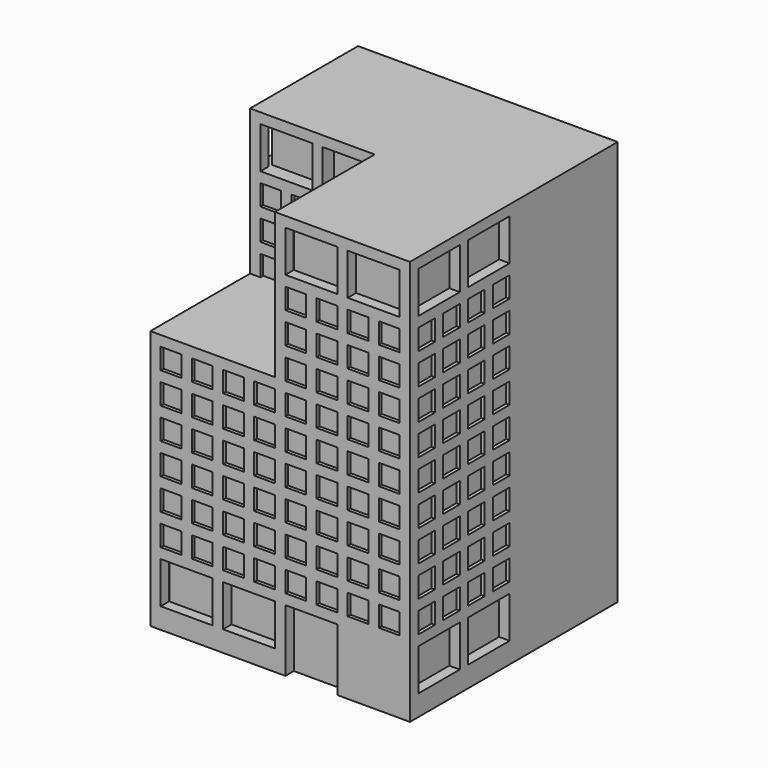
from build123d import *

# Parameters (mm, degrees)
F1_DEPTH     = 469.9
F2_W         = 225.552
F2_H         = 244.348
F3_DEPTH     = 281.94
F4_W         = 93.98
F4_H         = 75.184
F5_DEPTH     = 19.05
F4_W_2       = 37.592
F4_H_2       = 37.592
F6_DEPTH     = 6.35
F7_W         = 93.98
F7_H         = 75.184
F8_DEPTH     = 19.05
F7_W_2       = 187.96
F7_H_2       = 244.348
F7_W_3       = 37.592
F7_H_3       = 37.592
F9_DEPTH     = 6.35
F10_W        = 93.98
F10_H        = 75.184
F11_DEPTH    = 19.05
F10_W_2      = 37.592
F10_H_2      = 37.592
F12_DEPTH    = 6.35
F13_W        = 93.98
F13_H        = 75.184
F14_DEPTH    = 19.05
F13_W_2      = 37.592
F13_H_2      = 37.592
F13_W_3      = 187.96
F13_H_3      = 244.348
F15_DEPTH    = 6.35
F16_W        = 93.98
F16_H        = 75.184
F17_DEPTH    = 19.05
F16_W_2      = 37.592
F16_H_2      = 37.592
F18_DEPTH    = 6.35
F19_W        = 93.98
F19_H        = 75.184
F20_DEPTH    = 19.05
F21_DEPTH    = 224.028
F22_DEPTH    = 223.52
F19_W_2      = 37.592
F19_H_2      = 37.592
F20_FACE_W   = 93.726
F20_FACE_H   = 75.184
F20_FACE_W_2 = 93.98
F23_DEPTH    = 6.35
F24_DEPTH    = 18.796
F25_DEPTH    = 18.796


with BuildPart() as f1:
    # F0 (on Front) → F1 (new body)
    with BuildSketch(Plane.XZ):
        Polygon((109.2016026378, 21.9071136281), (109.2016026378, -466.788886372), (579.1016026378, -466.788886372), (579.1016026378, 303.847113628), (334.7536026378, 303.847113628), (334.7536026378, 21.9071136281), align=None)
    extrude(amount=F1_DEPTH)

    # F2 (on face) → F3 (join)
    with BuildSketch(Plane.XY.offset(21.907113628)):
        with Locations((221.9776026378, -122.174)):
            Rectangle(F2_W, F2_H)
    extrude(amount=F3_DEPTH)

    # F4 (on face) → F5 (cut)
    with BuildSketch(Plane.XZ.offset(469.9)):
        with Locations((400.5396026378, 228.663113628)):
            Rectangle(F4_W, F4_H)
        with Locations((513.3156026378, 228.663113628)):
            Rectangle(F4_W, F4_H)
        Polygon((447.5296026378, -335.216886372), (353.5496026378, -335.216886372), (353.5496026378, -410.400886372), (353.5496026378, -466.788886372), (447.5296026378, -466.788886372), (447.5296026378, -410.400886372), align=None)
        with Locations((287.7636026378, -372.808886372)):
            Rectangle(F4_W, F4_H)
        with Locations((174.9876026378, -372.808886372)):
            Rectangle(F4_W, F4_H)
    extrude(amount=-F5_DEPTH, mode=Mode.SUBTRACT)

    # F4 (on face) → F6 (cut)
    with BuildSketch(Plane.XZ.offset(469.9)):
        with Locations((174.9876026378, -372.808886372)):
            Rectangle(F4_W, F4_H)
        with Locations((287.7636026378, -372.808886372)):
            Rectangle(F4_W, F4_H)
        with Locations((541.5096026378, -297.624886372)):
            Rectangle(F4_W_2, F4_H_2)
        with Locations((541.5096026378, -241.236886372)):
            Rectangle(F4_W_2, F4_H_2)
        with Locations((541.5096026378, -184.848886372)):
            Rectangle(F4_W_2, F4_H_2)
        with Locations((541.5096026378, -128.460886372)):
            Rectangle(F4_W_2, F4_H_2)
        with Locations((541.5096026378, -72.072886372)):
            Rectangle(F4_W_2, F4_H_2)
        with Locations((541.5096026378, -15.684886372)):
            Rectangle(F4_W_2, F4_H_2)
        with Locations((485.1216026378, -297.624886372)):
            Rectangle(F4_W_2, F4_H_2)
        with Locations((485.1216026378, -241.236886372)):
            Rectangle(F4_W_2, F4_H_2)
        with Locations((485.1216026378, -184.848886372)):
            Rectangle(F4_W_2, F4_H_2)
        with Locations((485.1216026378, -128.460886372)):
            Rectangle(F4_W_2, F4_H_2)
        with Locations((485.1216026378, -72.072886372)):
            Rectangle(F4_W_2, F4_H_2)
        with Locations((485.1216026378, -15.684886372)):
            Rectangle(F4_W_2, F4_H_2)
        with Locations((428.7336026378, -297.624886372)):
            Rectangle(F4_W_2, F4_H_2)
        with Locations((428.7336026378, -241.236886372)):
            Rectangle(F4_W_2, F4_H_2)
        with Locations((428.7336026378, -184.848886372)):
            Rectangle(F4_W_2, F4_H_2)
        with Locations((428.7336026378, -128.460886372)):
            Rectangle(F4_W_2, F4_H_2)
        with Locations((428.7336026378, -72.072886372)):
            Rectangle(F4_W_2, F4_H_2)
        with Locations((428.7336026378, -15.684886372)):
            Rectangle(F4_W_2, F4_H_2)
        with Locations((372.3456026378, -297.624886372)):
            Rectangle(F4_W_2, F4_H_2)
        with Locations((372.3456026378, -241.236886372)):
            Rectangle(F4_W_2, F4_H_2)
        with Locations((372.3456026378, -184.848886372)):
            Rectangle(F4_W_2, F4_H_2)
        with Locations((372.3456026378, -128.460886372)):
            Rectangle(F4_W_2, F4_H_2)
        with Locations((372.3456026378, -72.072886372)):
            Rectangle(F4_W_2, F4_H_2)
        with Locations((372.3456026378, -15.684886372)):
            Rectangle(F4_W_2, F4_H_2)
        with Locations((315.9576026378, -297.624886372)):
            Rectangle(F4_W_2, F4_H_2)
        with Locations((315.9576026378, -241.236886372)):
            Rectangle(F4_W_2, F4_H_2)
        with Locations((315.9576026378, -184.848886372)):
            Rectangle(F4_W_2, F4_H_2)
        with Locations((315.9576026378, -128.460886372)):
            Rectangle(F4_W_2, F4_H_2)
        with Locations((315.9576026378, -72.072886372)):
            Rectangle(F4_W_2, F4_H_2)
        with Locations((315.9576026378, -15.684886372)):
            Rectangle(F4_W_2, F4_H_2)
        with Locations((259.5696026378, -297.624886372)):
            Rectangle(F4_W_2, F4_H_2)
        with Locations((259.5696026378, -241.236886372)):
            Rectangle(F4_W_2, F4_H_2)
        with Locations((259.5696026378, -184.848886372)):
            Rectangle(F4_W_2, F4_H_2)
        with Locations((259.5696026378, -128.460886372)):
            Rectangle(F4_W_2, F4_H_2)
        with Locations((259.5696026378, -72.072886372)):
            Rectangle(F4_W_2, F4_H_2)
        with Locations((259.5696026378, -15.684886372)):
            Rectangle(F4_W_2, F4_H_2)
        with Locations((203.1816026378, -297.624886372)):
            Rectangle(F4_W_2, F4_H_2)
        with Locations((203.1816026378, -241.236886372)):
            Rectangle(F4_W_2, F4_H_2)
        with Locations((203.1816026378, -184.848886372)):
            Rectangle(F4_W_2, F4_H_2)
        with Locations((203.1816026378, -128.460886372)):
            Rectangle(F4_W_2, F4_H_2)
        with Locations((203.1816026378, -72.072886372)):
            Rectangle(F4_W_2, F4_H_2)
        with Locations((203.1816026378, -15.684886372)):
            Rectangle(F4_W_2, F4_H_2)
        with Locations((146.7936026378, -297.624886372)):
            Rectangle(F4_W_2, F4_H_2)
        with Locations((146.7936026378, -241.236886372)):
            Rectangle(F4_W_2, F4_H_2)
        with Locations((146.7936026378, -184.848886372)):
            Rectangle(F4_W_2, F4_H_2)
        with Locations((146.7936026378, -128.460886372)):
            Rectangle(F4_W_2, F4_H_2)
        with Locations((146.7936026378, -72.072886372)):
            Rectangle(F4_W_2, F4_H_2)
        with Locations((146.7936026378, -15.684886372)):
            Rectangle(F4_W_2, F4_H_2)
        with Locations((513.3156026378, 228.663113628)):
            Rectangle(F4_W, F4_H)
        with Locations((400.5396026378, 228.663113628)):
            Rectangle(F4_W, F4_H)
        with Locations((541.5096026378, 40.703113628)):
            Rectangle(F4_W_2, F4_H_2)
        with Locations((541.5096026378, 97.091113628)):
            Rectangle(F4_W_2, F4_H_2)
        with Locations((541.5096026378, 153.479113628)):
            Rectangle(F4_W_2, F4_H_2)
        with Locations((485.1216026378, 40.703113628)):
            Rectangle(F4_W_2, F4_H_2)
        with Locations((485.1216026378, 97.091113628)):
            Rectangle(F4_W_2, F4_H_2)
        with Locations((485.1216026378, 153.479113628)):
            Rectangle(F4_W_2, F4_H_2)
        with Locations((428.7336026378, 40.703113628)):
            Rectangle(F4_W_2, F4_H_2)
        with Locations((428.7336026378, 97.091113628)):
            Rectangle(F4_W_2, F4_H_2)
        with Locations((428.7336026378, 153.479113628)):
            Rectangle(F4_W_2, F4_H_2)
        with Locations((372.3456026378, 40.703113628)):
            Rectangle(F4_W_2, F4_H_2)
        with Locations((372.3456026378, 97.091113628)):
            Rectangle(F4_W_2, F4_H_2)
        with Locations((372.3456026378, 153.479113628)):
            Rectangle(F4_W_2, F4_H_2)
    extrude(amount=-F6_DEPTH, mode=Mode.SUBTRACT)

    # F7 (on face) → F8 (cut)
    with BuildSketch(Plane(origin=(0, 0, 0), x_dir=(-1, 0, 0), z_dir=(0, 1, 0))):
        with Locations((-400.5396026378, 228.663113628)):
            Rectangle(F7_W, F7_H)
        with Locations((-287.7636026378, 228.663113628)):
            Rectangle(F7_W, F7_H)
        with Locations((-174.9876026378, 228.663113628)):
            Rectangle(F7_W, F7_H)
        with Locations((-400.5396026378, -372.8088863719)):
            Rectangle(F7_W, F7_H)
    extrude(amount=-F8_DEPTH, mode=Mode.SUBTRACT)

    # F7 (on face) → F9 (cut)
    with BuildSketch(Plane(origin=(0, 0, 0), x_dir=(-1, 0, 0), z_dir=(0, 1, 0))):
        with Locations((-240.7736026378, -344.614886372)):
            Rectangle(F7_W_2, F7_H_2)
        with Locations((-400.5396026378, -372.8088863719)):
            Rectangle(F7_W, F7_H)
        with Locations((-174.9876026378, 228.663113628)):
            Rectangle(F7_W, F7_H)
        with Locations((-287.7636026378, 228.663113628)):
            Rectangle(F7_W, F7_H)
        with Locations((-400.5396026378, 228.663113628)):
            Rectangle(F7_W, F7_H)
        with Locations((-146.7936026378, 153.479113628)):
            Rectangle(F7_W_3, F7_H_3)
        with Locations((-146.7936026378, 97.091113628)):
            Rectangle(F7_W_3, F7_H_3)
        with Locations((-146.7936026378, 40.703113628)):
            Rectangle(F7_W_3, F7_H_3)
        with Locations((-146.7936026378, -15.684886372)):
            Rectangle(F7_W_3, F7_H_3)
        with Locations((-146.7936026378, -72.072886372)):
            Rectangle(F7_W_3, F7_H_3)
        with Locations((-146.7936026378, -128.460886372)):
            Rectangle(F7_W_3, F7_H_3)
        with Locations((-146.7936026378, -184.848886372)):
            Rectangle(F7_W_3, F7_H_3)
        with Locations((-203.1816026378, 153.479113628)):
            Rectangle(F7_W_3, F7_H_3)
        with Locations((-203.1816026378, 97.091113628)):
            Rectangle(F7_W_3, F7_H_3)
        with Locations((-203.1816026378, 40.703113628)):
            Rectangle(F7_W_3, F7_H_3)
        with Locations((-203.1816026378, -15.684886372)):
            Rectangle(F7_W_3, F7_H_3)
        with Locations((-203.1816026378, -72.072886372)):
            Rectangle(F7_W_3, F7_H_3)
        with Locations((-203.1816026378, -128.460886372)):
            Rectangle(F7_W_3, F7_H_3)
        with Locations((-203.1816026378, -184.848886372)):
            Rectangle(F7_W_3, F7_H_3)
        with Locations((-259.5696026378, 153.479113628)):
            Rectangle(F7_W_3, F7_H_3)
        with Locations((-259.5696026378, 97.091113628)):
            Rectangle(F7_W_3, F7_H_3)
        with Locations((-259.5696026378, 40.703113628)):
            Rectangle(F7_W_3, F7_H_3)
        with Locations((-259.5696026378, -15.684886372)):
            Rectangle(F7_W_3, F7_H_3)
        with Locations((-259.5696026378, -72.072886372)):
            Rectangle(F7_W_3, F7_H_3)
        with Locations((-259.5696026378, -128.460886372)):
            Rectangle(F7_W_3, F7_H_3)
        with Locations((-259.5696026378, -184.848886372)):
            Rectangle(F7_W_3, F7_H_3)
        with Locations((-315.9576026378, 153.479113628)):
            Rectangle(F7_W_3, F7_H_3)
        with Locations((-315.9576026378, 97.091113628)):
            Rectangle(F7_W_3, F7_H_3)
        with Locations((-315.9576026378, 40.703113628)):
            Rectangle(F7_W_3, F7_H_3)
        with Locations((-315.9576026378, -15.684886372)):
            Rectangle(F7_W_3, F7_H_3)
        with Locations((-315.9576026378, -72.072886372)):
            Rectangle(F7_W_3, F7_H_3)
        with Locations((-315.9576026378, -128.460886372)):
            Rectangle(F7_W_3, F7_H_3)
        with Locations((-315.9576026378, -184.848886372)):
            Rectangle(F7_W_3, F7_H_3)
        with Locations((-372.3456026378, 153.479113628)):
            Rectangle(F7_W_3, F7_H_3)
        with Locations((-372.3456026378, 97.091113628)):
            Rectangle(F7_W_3, F7_H_3)
        with Locations((-372.3456026378, 40.703113628)):
            Rectangle(F7_W_3, F7_H_3)
        with Locations((-372.3456026378, -15.684886372)):
            Rectangle(F7_W_3, F7_H_3)
        with Locations((-372.3456026378, -72.072886372)):
            Rectangle(F7_W_3, F7_H_3)
        with Locations((-372.3456026378, -128.460886372)):
            Rectangle(F7_W_3, F7_H_3)
        with Locations((-372.3456026378, -184.848886372)):
            Rectangle(F7_W_3, F7_H_3)
        with Locations((-372.3456026378, -241.236886372)):
            Rectangle(F7_W_3, F7_H_3)
        with Locations((-372.3456026378, -297.624886372)):
            Rectangle(F7_W_3, F7_H_3)
        with Locations((-428.7336026378, 153.479113628)):
            Rectangle(F7_W_3, F7_H_3)
        with Locations((-428.7336026378, 97.091113628)):
            Rectangle(F7_W_3, F7_H_3)
        with Locations((-428.7336026378, 40.703113628)):
            Rectangle(F7_W_3, F7_H_3)
        with Locations((-428.7336026378, -15.684886372)):
            Rectangle(F7_W_3, F7_H_3)
        with Locations((-428.7336026378, -72.072886372)):
            Rectangle(F7_W_3, F7_H_3)
        with Locations((-428.7336026378, -128.460886372)):
            Rectangle(F7_W_3, F7_H_3)
        with Locations((-428.7336026378, -184.848886372)):
            Rectangle(F7_W_3, F7_H_3)
        with Locations((-428.7336026378, -241.236886372)):
            Rectangle(F7_W_3, F7_H_3)
        with Locations((-428.7336026378, -297.624886372)):
            Rectangle(F7_W_3, F7_H_3)
    extrude(amount=-F9_DEPTH, mode=Mode.SUBTRACT)

    # F10 (on face) → F11 (cut)
    with BuildSketch(Plane.YZ.offset(579.1016026378)):
        with Locations((-291.338, -372.808886372)):
            Rectangle(F10_W, F10_H)
        with Locations((-404.114, -372.808886372)):
            Rectangle(F10_W, F10_H)
        with Locations((-404.114, 228.663113628)):
            Rectangle(F10_W, F10_H)
        with Locations((-291.338, 228.663113628)):
            Rectangle(F10_W, F10_H)
    extrude(amount=-F11_DEPTH, mode=Mode.SUBTRACT)

    # F10 (on face) → F12 (cut)
    with BuildSketch(Plane.YZ.offset(579.1016026378)):
        with Locations((-432.308, -297.624886372)):
            Rectangle(F10_W_2, F10_H_2)
        with Locations((-432.308, -241.236886372)):
            Rectangle(F10_W_2, F10_H_2)
        with Locations((-432.308, -184.848886372)):
            Rectangle(F10_W_2, F10_H_2)
        with Locations((-432.308, -128.460886372)):
            Rectangle(F10_W_2, F10_H_2)
        with Locations((-432.308, -72.072886372)):
            Rectangle(F10_W_2, F10_H_2)
        with Locations((-432.308, -15.684886372)):
            Rectangle(F10_W_2, F10_H_2)
        with Locations((-432.308, 40.703113628)):
            Rectangle(F10_W_2, F10_H_2)
        with Locations((-432.308, 97.091113628)):
            Rectangle(F10_W_2, F10_H_2)
        with Locations((-432.308, 153.479113628)):
            Rectangle(F10_W_2, F10_H_2)
        with Locations((-375.92, -297.624886372)):
            Rectangle(F10_W_2, F10_H_2)
        with Locations((-375.92, -241.236886372)):
            Rectangle(F10_W_2, F10_H_2)
        with Locations((-375.92, -184.848886372)):
            Rectangle(F10_W_2, F10_H_2)
        with Locations((-375.92, -128.460886372)):
            Rectangle(F10_W_2, F10_H_2)
        with Locations((-375.92, -72.072886372)):
            Rectangle(F10_W_2, F10_H_2)
        with Locations((-375.92, -15.684886372)):
            Rectangle(F10_W_2, F10_H_2)
        with Locations((-375.92, 40.703113628)):
            Rectangle(F10_W_2, F10_H_2)
        with Locations((-375.92, 97.091113628)):
            Rectangle(F10_W_2, F10_H_2)
        with Locations((-375.92, 153.479113628)):
            Rectangle(F10_W_2, F10_H_2)
        with Locations((-319.532, -297.624886372)):
            Rectangle(F10_W_2, F10_H_2)
        with Locations((-319.532, -241.236886372)):
            Rectangle(F10_W_2, F10_H_2)
        with Locations((-319.532, -184.848886372)):
            Rectangle(F10_W_2, F10_H_2)
        with Locations((-319.532, -128.460886372)):
            Rectangle(F10_W_2, F10_H_2)
        with Locations((-319.532, -72.072886372)):
            Rectangle(F10_W_2, F10_H_2)
        with Locations((-319.532, -15.684886372)):
            Rectangle(F10_W_2, F10_H_2)
        with Locations((-319.532, 40.703113628)):
            Rectangle(F10_W_2, F10_H_2)
        with Locations((-319.532, 97.091113628)):
            Rectangle(F10_W_2, F10_H_2)
        with Locations((-319.532, 153.479113628)):
            Rectangle(F10_W_2, F10_H_2)
        with Locations((-263.144, -297.624886372)):
            Rectangle(F10_W_2, F10_H_2)
        with Locations((-263.144, -241.236886372)):
            Rectangle(F10_W_2, F10_H_2)
        with Locations((-263.144, -184.848886372)):
            Rectangle(F10_W_2, F10_H_2)
        with Locations((-263.144, -128.460886372)):
            Rectangle(F10_W_2, F10_H_2)
        with Locations((-263.144, -72.072886372)):
            Rectangle(F10_W_2, F10_H_2)
        with Locations((-263.144, -15.684886372)):
            Rectangle(F10_W_2, F10_H_2)
        with Locations((-263.144, 40.703113628)):
            Rectangle(F10_W_2, F10_H_2)
        with Locations((-263.144, 97.091113628)):
            Rectangle(F10_W_2, F10_H_2)
        with Locations((-263.144, 153.479113628)):
            Rectangle(F10_W_2, F10_H_2)
        with Locations((-291.338, 228.663113628)):
            Rectangle(F10_W, F10_H)
        with Locations((-404.114, 228.663113628)):
            Rectangle(F10_W, F10_H)
        with Locations((-404.114, -372.808886372)):
            Rectangle(F10_W, F10_H)
        with Locations((-291.338, -372.808886372)):
            Rectangle(F10_W, F10_H)
    extrude(amount=-F12_DEPTH, mode=Mode.SUBTRACT)

    # F13 (on face) → F14 (cut)
    with BuildSketch(Plane(origin=(109.2016026378, 0, 0), x_dir=(0, -1, 0), z_dir=(-1, 0, 0))):
        with Locations((65.786, 228.663113628)):
            Rectangle(F13_W, F13_H)
        with Locations((178.562, 228.663113628)):
            Rectangle(F13_W, F13_H)
        with Locations((291.338, -372.808886372)):
            Rectangle(F13_W, F13_H)
        with Locations((404.114, -372.808886372)):
            Rectangle(F13_W, F13_H)
    extrude(amount=-F14_DEPTH, mode=Mode.SUBTRACT)

    # F13 (on face) → F15 (cut)
    with BuildSketch(Plane(origin=(109.2016026378, 0, 0), x_dir=(0, -1, 0), z_dir=(-1, 0, 0))):
        with Locations((65.786, 228.663113628)):
            Rectangle(F13_W, F13_H)
        with Locations((178.562, 228.663113628)):
            Rectangle(F13_W, F13_H)
        with Locations((37.592, 153.479113628)):
            Rectangle(F13_W_2, F13_H_2)
        with Locations((37.592, 97.091113628)):
            Rectangle(F13_W_2, F13_H_2)
        with Locations((37.592, 40.703113628)):
            Rectangle(F13_W_2, F13_H_2)
        with Locations((37.592, -15.684886372)):
            Rectangle(F13_W_2, F13_H_2)
        with Locations((37.592, -72.072886372)):
            Rectangle(F13_W_2, F13_H_2)
        with Locations((37.592, -128.460886372)):
            Rectangle(F13_W_2, F13_H_2)
        with Locations((37.592, -184.848886372)):
            Rectangle(F13_W_2, F13_H_2)
        with Locations((93.98, 153.479113628)):
            Rectangle(F13_W_2, F13_H_2)
        with Locations((93.98, 97.091113628)):
            Rectangle(F13_W_2, F13_H_2)
        with Locations((93.98, 40.703113628)):
            Rectangle(F13_W_2, F13_H_2)
        with Locations((93.98, -15.684886372)):
            Rectangle(F13_W_2, F13_H_2)
        with Locations((93.98, -72.072886372)):
            Rectangle(F13_W_2, F13_H_2)
        with Locations((93.98, -128.460886372)):
            Rectangle(F13_W_2, F13_H_2)
        with Locations((93.98, -184.848886372)):
            Rectangle(F13_W_2, F13_H_2)
        with Locations((150.368, 153.479113628)):
            Rectangle(F13_W_2, F13_H_2)
        with Locations((150.368, 97.091113628)):
            Rectangle(F13_W_2, F13_H_2)
        with Locations((150.368, 40.703113628)):
            Rectangle(F13_W_2, F13_H_2)
        with Locations((150.368, -15.684886372)):
            Rectangle(F13_W_2, F13_H_2)
        with Locations((150.368, -72.072886372)):
            Rectangle(F13_W_2, F13_H_2)
        with Locations((150.368, -128.460886372)):
            Rectangle(F13_W_2, F13_H_2)
        with Locations((150.368, -184.848886372)):
            Rectangle(F13_W_2, F13_H_2)
        with Locations((206.756, 153.479113628)):
            Rectangle(F13_W_2, F13_H_2)
        with Locations((206.756, 97.091113628)):
            Rectangle(F13_W_2, F13_H_2)
        with Locations((206.756, 40.703113628)):
            Rectangle(F13_W_2, F13_H_2)
        with Locations((206.756, -15.684886372)):
            Rectangle(F13_W_2, F13_H_2)
        with Locations((206.756, -72.072886372)):
            Rectangle(F13_W_2, F13_H_2)
        with Locations((206.756, -128.460886372)):
            Rectangle(F13_W_2, F13_H_2)
        with Locations((206.756, -184.848886372)):
            Rectangle(F13_W_2, F13_H_2)
        with Locations((263.144, -15.684886372)):
            Rectangle(F13_W_2, F13_H_2)
        with Locations((263.144, -72.072886372)):
            Rectangle(F13_W_2, F13_H_2)
        with Locations((263.144, -128.460886372)):
            Rectangle(F13_W_2, F13_H_2)
        with Locations((263.144, -184.848886372)):
            Rectangle(F13_W_2, F13_H_2)
        with Locations((263.144, -241.236886372)):
            Rectangle(F13_W_2, F13_H_2)
        with Locations((319.532, -15.684886372)):
            Rectangle(F13_W_2, F13_H_2)
        with Locations((319.532, -72.072886372)):
            Rectangle(F13_W_2, F13_H_2)
        with Locations((319.532, -128.460886372)):
            Rectangle(F13_W_2, F13_H_2)
        with Locations((319.532, -184.848886372)):
            Rectangle(F13_W_2, F13_H_2)
        with Locations((319.532, -241.236886372)):
            Rectangle(F13_W_2, F13_H_2)
        with Locations((375.92, -15.684886372)):
            Rectangle(F13_W_2, F13_H_2)
        with Locations((375.92, -72.072886372)):
            Rectangle(F13_W_2, F13_H_2)
        with Locations((375.92, -128.460886372)):
            Rectangle(F13_W_2, F13_H_2)
        with Locations((375.92, -184.848886372)):
            Rectangle(F13_W_2, F13_H_2)
        with Locations((375.92, -241.236886372)):
            Rectangle(F13_W_2, F13_H_2)
        with Locations((432.308, -15.684886372)):
            Rectangle(F13_W_2, F13_H_2)
        with Locations((432.308, -72.072886372)):
            Rectangle(F13_W_2, F13_H_2)
        with Locations((432.308, -128.460886372)):
            Rectangle(F13_W_2, F13_H_2)
        with Locations((432.308, -184.848886372)):
            Rectangle(F13_W_2, F13_H_2)
        with Locations((432.308, -241.236886372)):
            Rectangle(F13_W_2, F13_H_2)
        with Locations((263.144, -297.624886372)):
            Rectangle(F13_W_2, F13_H_2)
        with Locations((319.532, -297.624886372)):
            Rectangle(F13_W_2, F13_H_2)
        with Locations((375.92, -297.624886372)):
            Rectangle(F13_W_2, F13_H_2)
        with Locations((432.308, -297.624886372)):
            Rectangle(F13_W_2, F13_H_2)
        with Locations((291.338, -372.808886372)):
            Rectangle(F13_W, F13_H)
        with Locations((404.114, -372.808886372)):
            Rectangle(F13_W, F13_H)
        with Locations((131.572, -344.614886372)):
            Rectangle(F13_W_3, F13_H_3)
    extrude(amount=-F15_DEPTH, mode=Mode.SUBTRACT)

    # F16 (on face) → F17 (cut)
    with BuildSketch(Plane(origin=(334.7536026378, 0, 0), x_dir=(0, -1, 0), z_dir=(-1, 0, 0))):
        with Locations((404.114, 228.663113628)):
            Rectangle(F16_W, F16_H)
        with Locations((291.338, 228.663113628)):
            Rectangle(F16_W, F16_H)
    extrude(amount=-F17_DEPTH, mode=Mode.SUBTRACT)

    # F16 (on face) → F18 (cut)
    with BuildSketch(Plane(origin=(334.7536026378, 0, 0), x_dir=(0, -1, 0), z_dir=(-1, 0, 0))):
        with Locations((263.144, 153.479113628)):
            Rectangle(F16_W_2, F16_H_2)
        with Locations((263.144, 97.091113628)):
            Rectangle(F16_W_2, F16_H_2)
        with Locations((263.144, 40.703113628)):
            Rectangle(F16_W_2, F16_H_2)
        with Locations((319.532, 40.703113628)):
            Rectangle(F16_W_2, F16_H_2)
        with Locations((319.532, 97.091113628)):
            Rectangle(F16_W_2, F16_H_2)
        with Locations((319.532, 153.479113628)):
            Rectangle(F16_W_2, F16_H_2)
        with Locations((375.92, 153.479113628)):
            Rectangle(F16_W_2, F16_H_2)
        with Locations((375.92, 97.091113628)):
            Rectangle(F16_W_2, F16_H_2)
        with Locations((375.92, 40.703113628)):
            Rectangle(F16_W_2, F16_H_2)
        with Locations((432.308, 40.703113628)):
            Rectangle(F16_W_2, F16_H_2)
        with Locations((432.308, 97.091113628)):
            Rectangle(F16_W_2, F16_H_2)
        with Locations((432.308, 153.479113628)):
            Rectangle(F16_W_2, F16_H_2)
        with Locations((404.114, 228.663113628)):
            Rectangle(F16_W, F16_H)
        with Locations((291.338, 228.663113628)):
            Rectangle(F16_W, F16_H)
    extrude(amount=-F18_DEPTH, mode=Mode.SUBTRACT)

    # F19 (on face) → F20 (cut)
    with BuildSketch(Plane.XZ.offset(244.348)):
        with Locations((174.9876026378, 228.663113628)):
            Rectangle(F19_W, F19_H)
        with Locations((287.7636026378, 228.663113628)):
            Rectangle(F19_W, F19_H)
    extrude(amount=-F20_DEPTH, mode=Mode.SUBTRACT)

    # F7 (on face) → F21 (cut)
    with BuildSketch(Plane(origin=(0, 0, 0), x_dir=(-1, 0, 0), z_dir=(0, 1, 0))):
        with Locations((-240.7736026378, -344.614886372)):
            Rectangle(F7_W_2, F7_H_2)
    extrude(amount=-F21_DEPTH, mode=Mode.SUBTRACT)

    # F13 (on face) → F22 (cut)
    with BuildSketch(Plane(origin=(109.2016026378, 0, 0), x_dir=(0, -1, 0), z_dir=(-1, 0, 0))):
        with Locations((131.572, -344.614886372)):
            Rectangle(F13_W_3, F13_H_3)
    extrude(amount=-F22_DEPTH, mode=Mode.SUBTRACT)

    # F19 (on face) + F20_face (on face) → F23 (cut)
    with BuildSketch(Plane.XZ.offset(244.348)):
        with Locations((146.7936026378, 153.479113628)):
            Rectangle(F19_W_2, F19_H_2)
        with Locations((203.1816026378, 153.479113628)):
            Rectangle(F19_W_2, F19_H_2)
        with Locations((259.5696026378, 153.479113628)):
            Rectangle(F19_W_2, F19_H_2)
        with Locations((315.9576026378, 153.479113628)):
            Rectangle(F19_W_2, F19_H_2)
        with Locations((315.9576026378, 97.091113628)):
            Rectangle(F19_W_2, F19_H_2)
        with Locations((259.5696026378, 97.091113628)):
            Rectangle(F19_W_2, F19_H_2)
        with Locations((203.1816026378, 97.091113628)):
            Rectangle(F19_W_2, F19_H_2)
        with Locations((146.7936026378, 97.091113628)):
            Rectangle(F19_W_2, F19_H_2)
        with Locations((146.7936026378, 40.703113628)):
            Rectangle(F19_W_2, F19_H_2)
        with Locations((203.1816026378, 40.703113628)):
            Rectangle(F19_W_2, F19_H_2)
        with Locations((259.5696026378, 40.703113628)):
            Rectangle(F19_W_2, F19_H_2)
        with Locations((315.9576026378, 40.703113628)):
            Rectangle(F19_W_2, F19_H_2)
    with BuildSketch(Plane(origin=(175.1146026378, -225.298, 228.663113628), x_dir=(1, 0, 0), z_dir=(0, -1, 0))):
        Rectangle(F20_FACE_W, F20_FACE_H)
        with Locations((112.649, 0)):
            Rectangle(F20_FACE_W_2, F20_FACE_H)
    extrude(amount=-F23_DEPTH, mode=Mode.SUBTRACT)

    # F24 (cut): faces of the model
    f24_faces = [f1.faces().sort_by_distance(p)[0] for p in [
        (380.5157896218, -269.5143760071, -466.788886372),
        (127.9976026378, -18.796, -466.788886372),
    ]]
    extrude(f24_faces, amount=-F24_DEPTH, mode=Mode.SUBTRACT)

    # F25 (cut): a face of the model
    f25_faces = [f1.faces().sort_by_distance(p)[0] for p in [
        (380.7276026378, -198.374, 303.847113628),
    ]]
    extrude(f25_faces, amount=-F25_DEPTH, mode=Mode.SUBTRACT)


solid = f1.part
